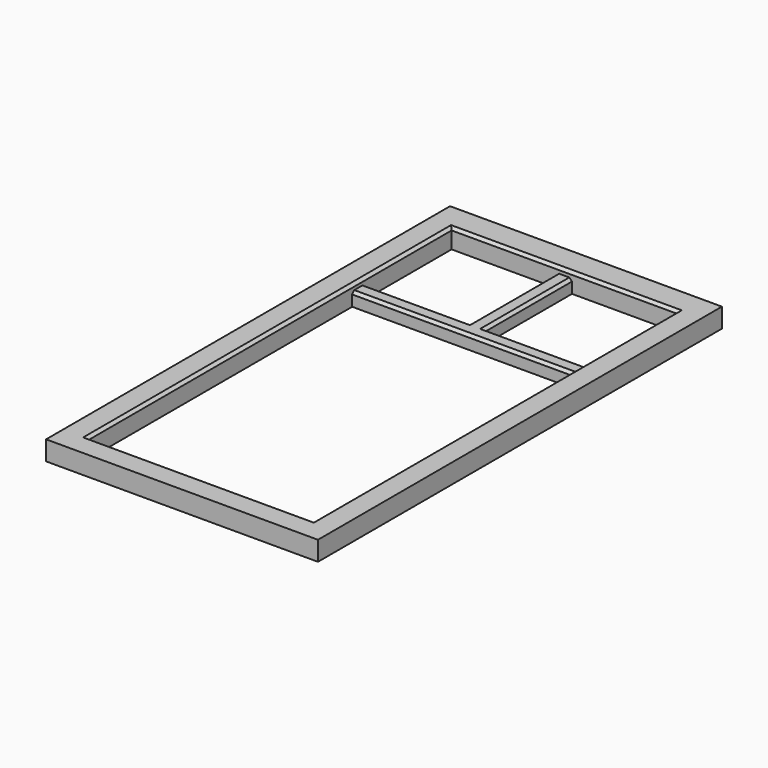
from build123d import *

# Parameters (mm, degrees)
F0_W      = 700
F0_H      = 1300
F1_DEPTH  = 50
F2_DEPTH  = 35
F3_SIZE   = 7
F3_2_SIZE = 7


# Not quite as in the source:
# - a feature names something its author has since deleted; it is built from what else it names


with BuildPart() as f1:
    # F0 (on Top) → F1 (new body)
    with BuildSketch(Plane.XY):
        with Locations((28.3141621128, 115.2047318473)):
            Rectangle(F0_W, F0_H)
        Polygon((-261.6858378872, 415.2047318473), (-261.6858378872, 695.2047318473), (8.3141621128, 695.2047318473), (48.3141621128, 695.2047318473), (318.3141621128, 695.2047318473), (318.3141621128, 415.2047318473), (318.3141621128, 375.2047318473), (318.3141621128, -474.7952681527), (-261.6858378872, -474.7952681527), (-261.6858378872, 375.2047318473), align=None, mode=Mode.SUBTRACT)
    extrude(amount=F1_DEPTH)

    # F3
    f3_edges = [f1.edges().sort_by_distance(p)[0] for p in [
        (-261.685838, 110.204732, 50),
        (318.314162, 110.204732, 50),
        (28.314162, 695.204732, 50),
        (28.314162, -474.795268, 50),
    ]]
    chamfer(f3_edges, length=F3_SIZE)


with BuildPart() as f2:
    # F0 (on Top) → F2 (new body)
    with BuildSketch(Plane.XY):
        Polygon((48.3141621128, 695.2047318473), (8.3141621128, 695.2047318473), (8.3141621128, 415.2047318473), (-261.6858378872, 415.2047318473), (-261.6858378872, 375.2047318473), (318.3141621128, 375.2047318473), (318.3141621128, 415.2047318473), (48.3141621128, 415.2047318473), align=None)
    extrude(amount=F2_DEPTH)

    # F3#2
    f3_2_edges = [f2.edges().sort_by_distance(p)[0] for p in [
        (8.314162, 555.204732, 35),
        (48.314162, 555.204732, 35),
        (-126.685838, 415.204732, 35),
        (183.314162, 415.204732, 35),
        (28.314162, 375.204732, 35),
    ]]
    chamfer(f3_2_edges, length=F3_2_SIZE)


solid = Compound([f1.part, f2.part])
